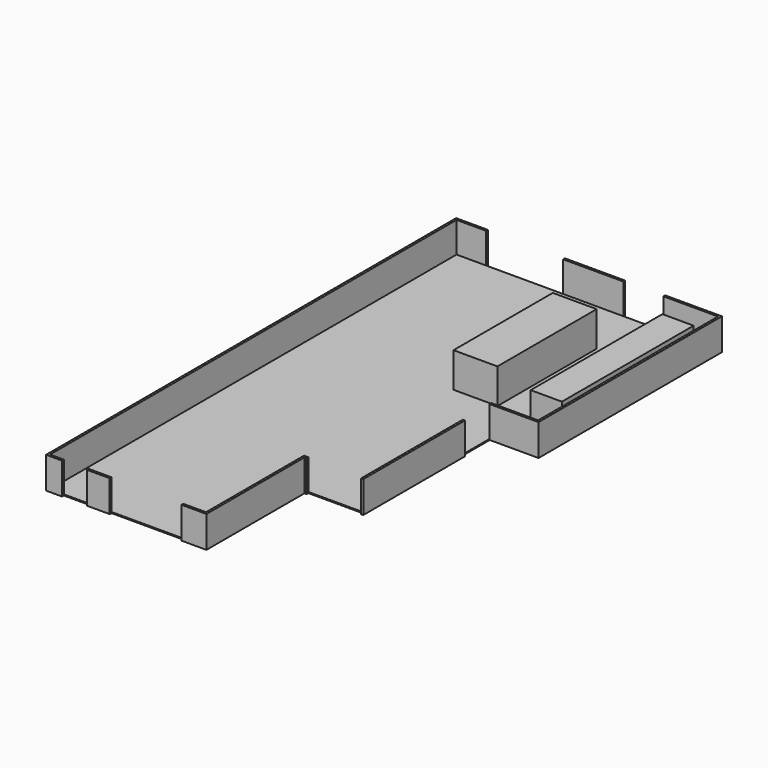
from build123d import *

# Parameters (mm, degrees)
F0_W          = 1007.6858997345
F0_H          = 2846.6820716858
F1_DEPTH      = 25
F0_W_2        = 50
F0_H_2        = 11660
F0_W_3        = 680.754840374
F0_H_3        = 50
F0_W_4        = 525.554060936
F0_W_5        = 1380.6488513947
F2_DEPTH      = 700
F2_DEPTH_BACK = 25
F0_W_6        = 716.5780067444
F0_H_4        = 3777.3280143738
F3_DEPTH      = 800
F3_DEPTH_BACK = 25


with BuildPart() as f1:
    # F0 (on Top) → F1 (new body)
    with BuildSketch(Plane.XY):
        Polygon((0, 11660), (0, 0), (315.7672286034, 0), (884.3851089478, 0), (1409.9391698837, 0), (3058.6225986481, 0), (3580, 0), (3580, 2810), (3630, 2810), (3680, 2810), (4930, 2810), (4930, 5679.7533035278), (4930, 6450), (4930, 6500), (5082.5057029724, 6500), (6000, 6500), (6000, 7182.6367378235), (5283.4219932556, 7182.6367378235), (5283.4219932556, 10959.9647521973), (6000, 10959.9647521973), (6000, 11660), (4745.2807426453, 11660), (3829.149723053, 11660), (2448.5008716583, 11660), (680.754840374, 11660), align=None)
        with Locations((3739.4448518753, 8952.6889324188)):
            Rectangle(F0_W, F0_H, mode=Mode.SUBTRACT)
    extrude(amount=-F1_DEPTH)

    # F0 (on Top) → F2 (join, two sides)
    with BuildSketch(Plane.XY) as f2_sk:
        with Locations((-25, 5830)):
            Rectangle(F0_W_2, F0_H_2)
        Polygon((315.7672286034, 0), (0, 0), (-50, 0), (-50, -50), (315.7672286034, -50), align=None)
        with Locations((340.377420187, 11685)):
            Rectangle(F0_W_3, F0_H_3)
        with Locations((-25, 11685)):
            Rectangle(F0_W_2, F0_H_3)
        with Locations((1147.1621394157, -25)):
            Rectangle(F0_W_4, F0_H_3)
        with Locations((3138.8252973557, 11685)):
            Rectangle(F0_W_5, F0_H_3)
        Polygon((3580, 0), (3058.6225986481, 0), (3058.6225986481, -50), (3630, -50), (3630, 0), align=None)
        Polygon((4745.2807426453, 11710), (4745.2807426453, 11660), (6000, 11660), (6050, 11660), (6050, 11710), align=None)
        Polygon((3580, 2810), (3580, 0), (3630, 0), (3630, 2760), (3630, 2810), align=None)
        Polygon((6050, 11660), (6000, 11660), (6000, 10959.9647521973), (6000, 7182.6367378235), (6000, 6500), (6000, 6450), (6050, 6450), align=None)
        with Locations((3655, 2785)):
            Rectangle(F0_W_2, F0_H_3)
        Polygon((6000, 6450), (6000, 6500), (5082.5057029724, 6500), (4930, 6500), (4930, 6450), align=None)
        Polygon((4930, 5679.7533035278), (4930, 2810), (4930, 2760), (4980, 2760), (4980, 5679.7533035278), align=None)
    extrude(amount=F2_DEPTH)
    extrude(f2_sk.sketch, amount=-F2_DEPTH_BACK)

    # F0 (on Top) → F3 (join, two sides)
    with BuildSketch(Plane.XY) as f3_sk:
        with Locations((3739.4448518753, 8952.6889324188)):
            Rectangle(F0_W, F0_H)
        with Locations((5641.7109966278, 9071.3007450104)):
            Rectangle(F0_W_6, F0_H_4)
    extrude(amount=F3_DEPTH)
    extrude(f3_sk.sketch, amount=-F3_DEPTH_BACK)


solid = f1.part
